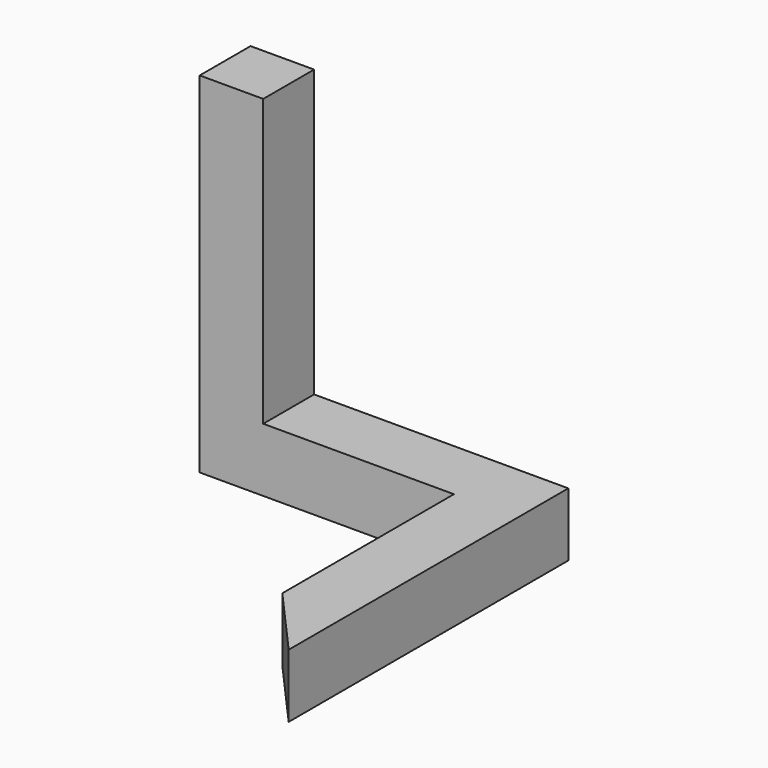
from build123d import *

# Parameters (mm, degrees)
F0_W     = 10
F0_H     = 10
F1_DEPTH = 50
F2_W     = 10
F2_H     = 10
F3_DEPTH = 50
F4_W     = 10
F4_H     = 10
F5_DEPTH = 50
F6_SIZE2 = 9.99999
F6_SIZE  = 11.24999


# Not quite as in the source:
# - a fillet or chamfer is up to 0.001 mm smaller than in the source, because OpenCascade refuses the exact size


with BuildPart() as f1:
    # F0 (on Right) → F1 (new body)
    with BuildSketch(Plane.YZ):
        Rectangle(F0_W, F0_H)
    extrude(amount=F1_DEPTH)

    # F2 (on Top) → F3 (join)
    with BuildSketch(Plane.XY):
        with Locations((5, 0)):
            Rectangle(F2_W, F2_H)
    extrude(amount=F3_DEPTH)

    # F4 (on Front) → F5 (join)
    with BuildSketch(Plane.XZ):
        with Locations((45, 0)):
            Rectangle(F4_W, F4_H)
    extrude(amount=F5_DEPTH)

    # F6 (size 11.25 and 10 in the source; OpenCascade refuses exactly that, so slightly less here)
    f6_edges = [f1.edges().sort_by_distance(p)[0] for p in [
        (40, -50, 0),
    ]]
    f6_side = f1.faces().sort_by_distance((40, -27.5, 0))[0]
    chamfer(f6_edges, length=F6_SIZE, length2=F6_SIZE2, reference=f6_side)


solid = f1.part
